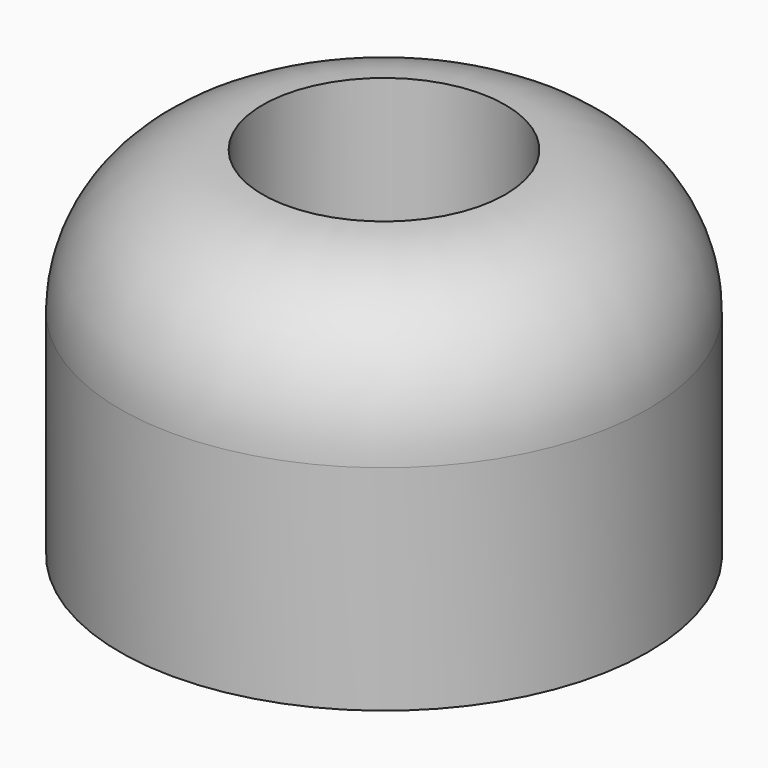
from build123d import *

# Parameters (mm, degrees)
F0_R         = 9.4039721792
F1_DEPTH     = 12.7
F5_R         = 5.08
F6_DEPTH     = 8.89
F7_TEXT_SIZE = 4.2004644961
F8_DEPTH     = 2.54


# Not quite as in the source:
# - the program builds the solid bodies; features that only make, move or delete a surface that nothing else refers to are left out
# - Text() gives the source's letters only with a copy of the font that has no kerning and outlines rounded to 1/6400 em; it was checked with that copy


with BuildPart() as f1:
    # F0 (on Top) → F1 (new body)
    with BuildSketch(Plane.XY):
        Circle(F0_R)
    extrude(amount=F1_DEPTH)

    # F5
    f5_edges = [f1.edges().sort_by_distance(p)[0] for p in [
        (-9.403972, 0, 12.7),
    ]]
    fillet(f5_edges, radius=F5_R)

    # F6 (cut): a face of the model
    f6_faces = [f1.faces().sort_by_distance(p)[0] for p in [
        (0, 0, 12.7),
    ]]
    extrude(f6_faces, amount=-F6_DEPTH, mode=Mode.SUBTRACT)

    # F7 (on face) → F8 (join)
    with BuildSketch(Plane.XY.offset(3.81)):
        with Locations((-3.8918603168, -1.5695564216)):
            Text('KRB', F7_TEXT_SIZE, font='Open Sans', text_align=(TextAlign.LEFT, TextAlign.BOTTOM))
    extrude(amount=F8_DEPTH)


solid = f1.part
